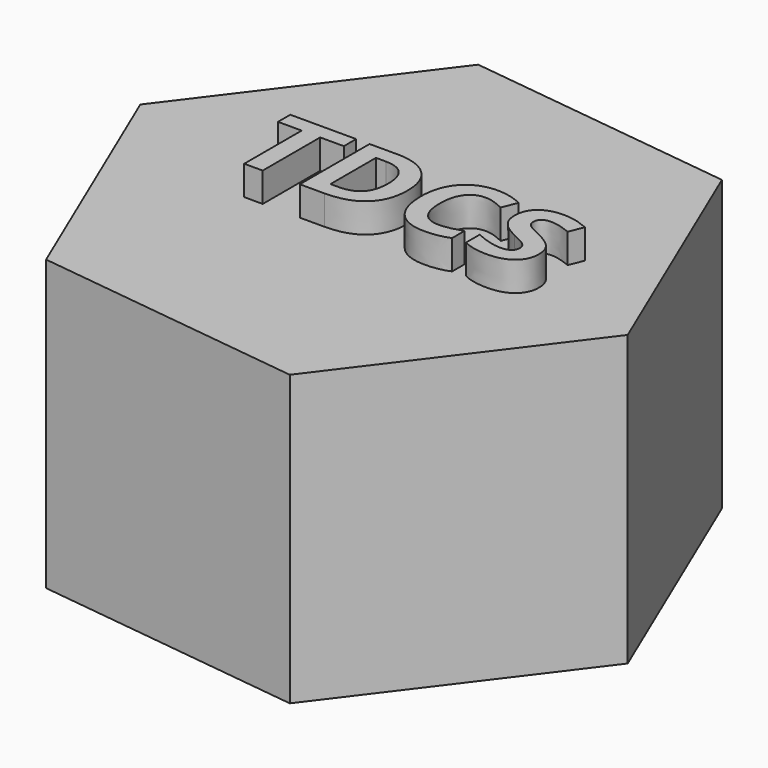
from build123d import *

# Parameters (mm, degrees)
F1_DEPTH     = 47.498
F2_TEXT_SIZE = 20.0579924733
F3_DEPTH     = 4.826


# Not quite as in the source:
# - Text() gives the source's letters only with a copy of the font that has no kerning and outlines rounded to 1/6400 em; it was checked with that copy


with BuildPart() as f1:
    # F0 (on Top) → F1 (new body)
    with BuildSketch(Plane.XY):
        Polygon((-16.2166229822, -15.1906218316), (10.7046392187, 20.5140383851), (-6.7558724619, 61.6808654614), (-51.1376463436, 67.143032321), (-78.0589085445, 31.4383721043), (-60.5983968638, -9.728454972), align=None)
    extrude(amount=F1_DEPTH)

    # F2 (on face) → F3 (join)
    with BuildSketch(Plane.XY.offset(47.498)):
        with Locations((-55.88, 19.6747553987)):
            Text('TDCS', F2_TEXT_SIZE, font='Open Sans', font_style=FontStyle.BOLD, text_align=(TextAlign.LEFT, TextAlign.BOTTOM))
    extrude(amount=F3_DEPTH)


solid = f1.part
